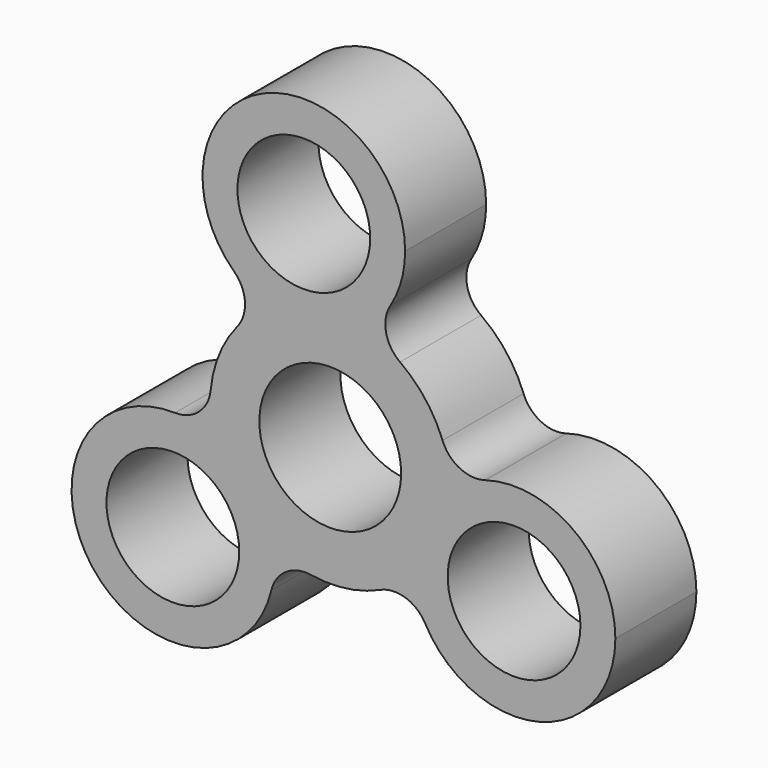
from build123d import *

# Parameters (mm, degrees)
F0_R     = 16.384259
F0_R_2   = 17.5
F1_DEPTH = 12.5
F2_R     = 8.649199


with BuildPart() as f1:
    # F0 (on Front) → F1 (new body, symmetric)
    with BuildSketch(Plane.XZ):
        with BuildLine():
            ThreePointArc((-15.490652, 25.284254), (-3.942062, 29.38901), (8.280022, 28.472707))
            ThreePointArc((8.280022, 28.472707), (15.783572, 37.329275), (18.478414, 48.619974))
            ThreePointArc((18.478414, 48.619974), (-20.677386, 69.226122), (-15.490652, 25.284254))
        make_face()
        with Locations((-6.521586, 48.619974)):
            Circle(F0_R, mode=Mode.SUBTRACT)
        with BuildLine():
            ThreePointArc((20.518076, -21.407063), (22.246679, -9.151388), (29.642132, 0.773171))
            ThreePointArc((29.642132, 0.773171), (23.480598, 18.108431), (8.280022, 28.472707))
            ThreePointArc((8.280022, 28.472707), (-3.198005, 23.841883), (-15.490652, 25.284254))
            ThreePointArc((-15.490652, 25.284254), (-27.422661, 11.280579), (-28.798098, -7.065644))
            ThreePointArc((-28.798098, -7.065644), (-19.048674, -14.690495), (-14.15148, -26.057425))
            ThreePointArc((-14.15148, -26.057425), (3.942062, -29.38901), (20.518076, -21.407063))
        make_face()
        Circle(F0_R_2, mode=Mode.SUBTRACT)
        with BuildLine():
            ThreePointArc((-15.490652, 25.284254), (-3.198005, 23.841883), (8.280022, 28.472707))
            ThreePointArc((8.280022, 28.472707), (-3.942062, 29.38901), (-15.490652, 25.284254))
        make_face()
        with BuildLine():
            ThreePointArc((-13.84534, -29.957847), (-13.921992, -28.001638), (-14.15148, -26.057425))
            ThreePointArc((-14.15148, -26.057425), (-23.480598, -18.108431), (-28.798098, -7.065644))
            ThreePointArc((-28.798098, -7.065644), (-59.775952, -43.629331), (-13.84534, -29.957847))
        make_face()
        with Locations((-38.84534, -29.957847)):
            Circle(F0_R, mode=Mode.SUBTRACT)
        with BuildLine():
            ThreePointArc((29.642132, 0.773171), (29.649693, 0.386619), (29.652214, 0))
            ThreePointArc((29.652214, 0), (27.273249, -11.637169), (20.518076, -21.407063))
            ThreePointArc((20.518076, -21.407063), (46.741473, -43.624312), (70.366926, -18.662128))
            ThreePointArc((70.366926, -18.662128), (56.134473, 3.900229), (29.642132, 0.773171))
        make_face()
        with Locations((45.366926, -18.662128)):
            Circle(F0_R, mode=Mode.SUBTRACT)
        with BuildLine():
            ThreePointArc((20.518076, -21.407063), (27.273249, -11.637169), (29.652214, 0))
            ThreePointArc((29.652214, 0), (29.649693, 0.386619), (29.642132, 0.773171))
            ThreePointArc((29.642132, 0.773171), (22.246679, -9.151388), (20.518076, -21.407063))
        make_face()
        with BuildLine():
            ThreePointArc((-28.798098, -7.065644), (-23.480598, -18.108431), (-14.15148, -26.057425))
            ThreePointArc((-14.15148, -26.057425), (-19.048674, -14.690495), (-28.798098, -7.065644))
        make_face()
    extrude(amount=F1_DEPTH, both=True)

    # F2
    f2_edges = [f1.edges().sort_by_distance(p)[0] for p in [
        (-28.798098, 0, -7.065644),
        (-15.490652, 0, 25.284254),
        (-14.15148, 0, -26.057425),
        (20.518076, 0, -21.407063),
        (8.280022, 0, 28.472707),
        (29.642132, 0, 0.773171),
    ]]
    fillet(f2_edges, radius=F2_R)


solid = f1.part
